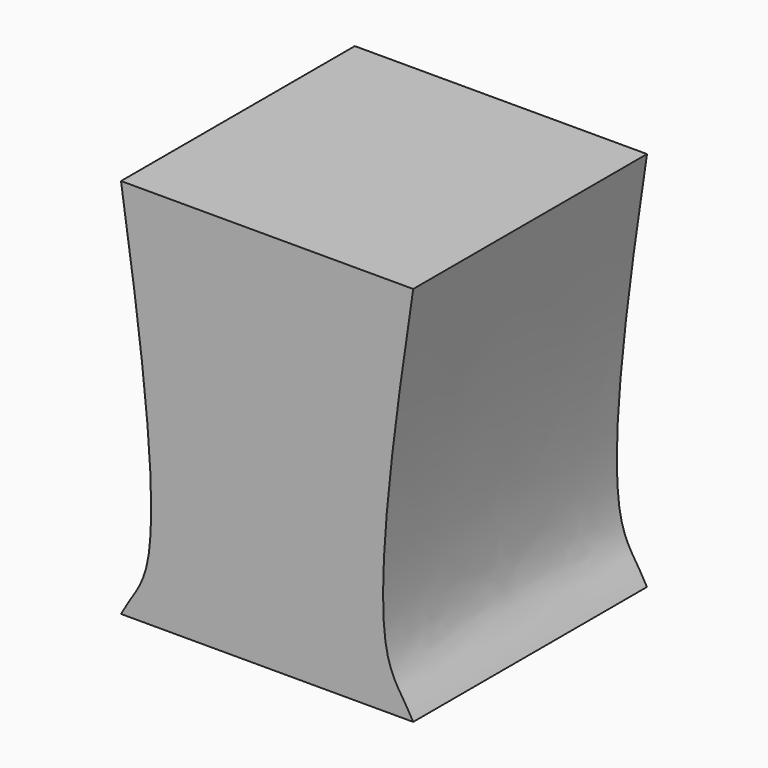
from build123d import *

# Parameters (mm, degrees)
F1_DEPTH = 115
F3_DEPTH = 65


# Not quite as in the source:
# - the dataset's text gives a spline's control points without its knots; the knots are read off the source's solid


with BuildPart() as f1:
    # F0 (on Front) → F1 (new body)
    with BuildSketch(Plane.XZ):
        with BuildLine():
            Line((-82.6327902788, 64.0317254593), (-197.6327902788, 64.0317254593))
            add(Edge.make_bspline(
                [(-197.6327902788, 64.0317254593), (-190.1866329645, 14.810095012), (-179.0788138277, -66.1737912972), (-193.7482136921, -78.4307880412), (-197.6327902788, -85.9682745407)],
                knots=[0, 0, 0, 0, 0.7018083927, 1, 1, 1, 1], degree=3))
            Line((-197.6327902788, -85.9682745407), (-82.6327902788, -85.9682745407))
            add(Edge.make_bspline(
                [(-82.6327902788, 64.0317254593), (-90.0789475931, 14.810095012), (-101.1867667298, -66.1737912972), (-86.5173668655, -78.4307880412), (-82.6327902788, -85.9682745407)],
                knots=[0, 0, 0, 0, 0.7018083927, 1, 1, 1, 1], degree=3))
        make_face()
    extrude(amount=F1_DEPTH)

    # F2 (on Right) → F3 (cut, symmetric)
    with BuildSketch(Plane.YZ):
        with BuildLine():
            add(Edge.make_bspline(
                [(-115, 64.0317254593), (-107.5538426857, 14.810095012), (-96.446023549, -66.1737912972), (-111.1154234133, -78.4307880412), (-115, -85.9682745407)],
                knots=[0, 0, 0, 0, 0.7018083927, 1, 1, 1, 1], degree=3))
            Line((-115, 64.0317254593), (-115, -85.9682745407))
        make_face()
        with BuildLine():
            Line((0, -85.9682745407), (0, 64.0317254593))
            add(Edge.make_bspline(
                [(0, 64.0317254593), (-7.4461573143, 14.810095012), (-18.553976451, -66.1737912972), (-3.8845765867, -78.4307880412), (0, -85.9682745407)],
                knots=[0, 0, 0, 0, 0.7018083927, 1, 1, 1, 1], degree=3))
        make_face()
    extrude(amount=F3_DEPTH, both=True, mode=Mode.SUBTRACT)


solid = f1.part
